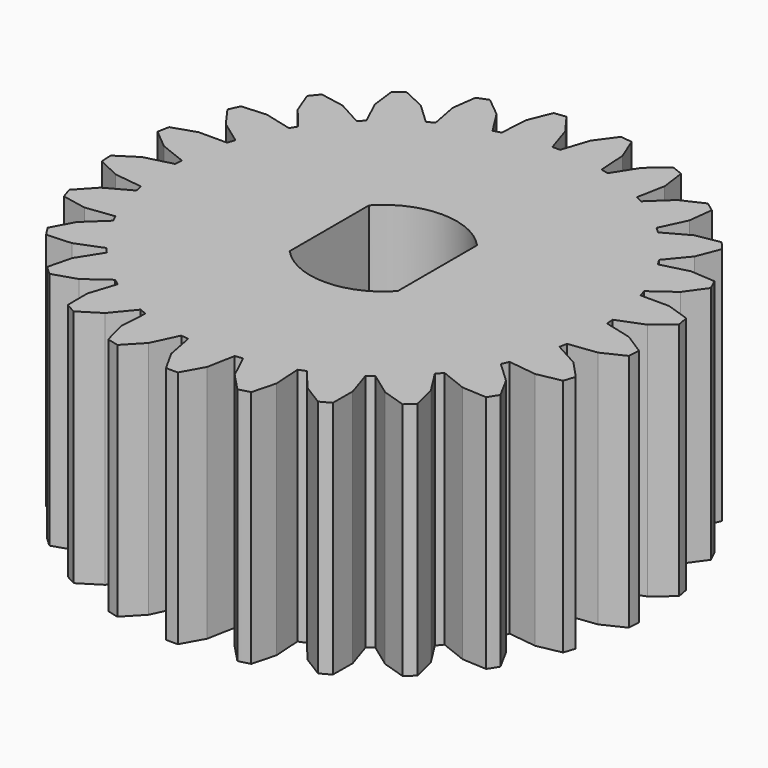
from build123d import *

# Parameters (mm, degrees)
F0_R     = 6.85
F1_DEPTH = 6.2
F3_DEPTH = 25


with BuildPart() as f1:
    # F0 (on Top) → F1 (new body)
    with BuildSketch(Plane.XY):
        Circle(F0_R)
        with BuildLine():
            ThreePointArc((1.4, -1.2845232579), (0, -1.9), (-1.4, -1.2845232579))
            Line((-1.4, -1.2845232579), (-1.4, 1.2845232579))
            ThreePointArc((-1.4, 1.2845232579), (0, 1.9), (1.4, 1.2845232579))
            Line((1.4, 1.2845232579), (1.4, -1.2845232579))
        make_face(mode=Mode.SUBTRACT)
    extrude(amount=F1_DEPTH)

    # F2 (on face) → F3 (cut)
    with BuildSketch(Plane.XY.offset(6.2)):
        with BuildLine():
            Line((0.3280050893, 6.3), (0.7057770525, 6.8135437734))
            ThreePointArc((0.7057770525, 6.8135437734), (0, 6.85), (-0.7057770525, 6.8135437734))
            Line((-0.7057770525, 6.8135437734), (-0.3280050893, 6.3))
            Line((-0.3280050893, 6.3), (-0.1, 5.5982724904))
            ThreePointArc((-0.1, 5.5982724904), (0.0002198008, 5.5998651199), (0.100452053, 5.5996637666))
            Line((0.100452053, 5.5996637666), (0.3280050893, 6.3))
        make_face()
        with BuildLine():
            ThreePointArc((-1.0108556636, 6.7750033821), (-1.7035257271, 6.6347946537), (-2.3780632008, 6.423964151))
            Line((-2.3780632008, 6.423964151), (-1.8844464954, 6.0205023665))
            Line((-1.8844464954, 6.0205023665), (-1.4890920701, 5.3975234769))
            ThreePointArc((-1.4890920701, 5.3975234769), (-1.3924169295, 5.4239897219), (-1.2952835832, 5.4487214421))
            Line((-1.2952835832, 5.4487214421), (-1.2490460829, 6.1836454637))
            Line((-1.2490460829, 6.1836454637), (-1.0108556636, 6.7750033821))
        make_face()
        with BuildLine():
            ThreePointArc((-2.6639726008, 6.3107646115), (-3.3000126676, 6.0027007583), (-3.9009268922, 5.6307432353))
            Line((-3.9009268922, 5.6307432353), (-3.3224811976, 5.3627144274))
            Line((-3.3224811976, 5.3627144274), (-2.7846190089, 4.8576282126))
            ThreePointArc((-2.7846190089, 4.8576282126), (-2.6975629831, 4.9073051017), (-2.6096317882, 4.9554159103))
            Line((-2.6096317882, 4.9554159103), (-2.747615096, 5.6787497411))
            Line((-2.747615096, 5.6787497411), (-2.6639726008, 6.3107646115))
        make_face()
        with BuildLine():
            ThreePointArc((-4.149702342, 5.4499972911), (-4.6891476756, 4.9934350978), (-5.1786810004, 4.4837220137))
            Line((-5.1786810004, 4.4837220137), (-4.5517521871, 4.3679674182))
            Line((-4.5517521871, 4.3679674182), (-3.9051780943, 4.0125103027))
            ThreePointArc((-3.9051780943, 4.0125103027), (-3.8332112335, 4.0822764541), (-3.7600072304, 4.1507433722))
            Line((-3.7600072304, 4.1507433722), (-4.0735413477, 4.8170372873))
            Line((-4.0735413477, 4.8170372873), (-4.149702342, 5.4499972911))
        make_face()
        with BuildLine():
            ThreePointArc((-5.3746910235, 4.2467865972), (-5.7836462897, 3.6704135456), (-6.1310395355, 3.054972048))
            Line((-6.1310395355, 3.054972048), (-5.4950198464, 3.0987649518))
            Line((-5.4950198464, 3.0987649518), (-4.7803604777, 2.9152716134))
            ThreePointArc((-4.7803604777, 2.9152716134), (-4.7280047246, 3.0007433634), (-4.6741275899, 3.0852643626))
            Line((-4.6741275899, 3.0852643626), (-5.143512015, 3.6526526649))
            Line((-5.143512015, 3.6526526649), (-5.3746910235, 4.2467865972))
        make_face()
        with BuildLine():
            ThreePointArc((-6.2619681013, 2.7767346827), (-6.5147371366, 2.1167664115), (-6.6981623082, 1.4342669531))
            Line((-6.6981623082, 1.4342669531), (-6.0930151995, 1.6348556871))
            Line((-6.0930151995, 1.6348556871), (-5.3551752314, 1.6348556871))
            ThreePointArc((-5.3551752314, 1.6348556871), (-5.3257202904, 1.7306625312), (-5.2945553228, 1.8259268463))
            Line((-5.2945553228, 1.8259268463), (-5.8902969058, 2.2587584421))
            Line((-5.8902969058, 2.2587584421), (-6.2619681013, 2.7767346827))
        make_face()
        with BuildLine():
            ThreePointArc((-6.7557826934, 1.1322103161), (-6.8364830897, 0.4301150588), (-6.844414909, -0.2765584093))
            Line((-6.844414909, -0.2765584093), (-6.3081639991, 0.0682224269))
            Line((-6.3081639991, 0.0682224269), (-5.5935046304, 0.2517157653))
            ThreePointArc((-5.5935046304, 0.2517157653), (-5.5888012638, 0.3518378072), (-5.5823066727, 0.451859631))
            Line((-5.5823066727, 0.451859631), (-6.2669727791, 0.7229381192))
            Line((-6.2669727791, 0.7229381192), (-6.7557826934, 1.1322103161))
        make_face()
        with BuildLine():
            ThreePointArc((-6.8251066128, -0.5834549887), (-6.7286676675, -1.2835620049), (-6.560607749, -1.9700065898))
            Line((-6.560607749, -1.9700065898), (-6.1269476548, -1.5026974992))
            Line((-6.1269476548, -1.5026974992), (-5.480373562, -1.1472403837))
            ThreePointArc((-5.480373562, -1.1472403837), (-5.5007172996, -1.0490941802), (-5.5193011641, -0.9505995868))
            Line((-5.5193011641, -0.9505995868), (-6.2498717044, -0.8583070645))
            Line((-6.2498717044, -0.8583070645), (-6.8251066128, -0.5834549887))
        make_face()
        with BuildLine():
            ThreePointArc((-6.4655839828, -2.2624596708), (-6.1980653094, -2.9165881472), (-5.8645734759, -3.539672011))
            Line((-5.8645734759, -3.539672011), (-5.560752656, -2.979197415))
            Line((-5.560752656, -2.979197415), (-5.0228904672, -2.4741112002))
            ThreePointArc((-5.0228904672, -2.4741112002), (-5.0670030372, -2.3841077219), (-5.1094976647, -2.2933291365))
            Line((-5.1094976647, -2.2933291365), (-5.8400682051, -2.3856216588))
            Line((-5.8400682051, -2.3856216588), (-6.4655839828, -2.2624596708))
        make_face()
        with BuildLine():
            ThreePointArc((-5.6998049323, -3.799305691), (-5.278015713, -4.3663543298), (-4.800046483, -4.8869268218))
            Line((-4.800046483, -4.8869268218), (-4.6451551168, -4.2685034004))
            Line((-4.6451551168, -4.2685034004), (-4.2498006916, -3.6455245108))
            ThreePointArc((-4.2498006916, -3.6455245108), (-4.3149103389, -3.5693190073), (-4.3786456357, -3.4919603822))
            Line((-4.3786456357, -3.4919603822), (-5.0633117421, -3.7630388704))
            Line((-5.0633117421, -3.7630388704), (-5.6998049323, -3.799305691))
        make_face()
        with BuildLine():
            ThreePointArc((-4.5758861756, -5.0974273617), (-4.0263289782, -5.5417664115), (-3.4339149162, -5.9271180475))
            Line((-3.4339149162, -5.9271180475), (-3.437685398, -5.2896036187))
            Line((-3.437685398, -5.2896036187), (-3.2096803087, -4.5878761091))
            ThreePointArc((-3.2096803087, -4.5878761091), (-3.2916959548, -4.5302568525), (-3.3726671978, -4.4711789146))
            Line((-3.3726671978, -4.4711789146), (-3.9684087809, -4.9040105104))
            Line((-3.9684087809, -4.9040105104), (-4.5758861756, -5.0974273617))
        make_face()
        with BuildLine():
            ThreePointArc((-3.1644476615, -6.0752589243), (-2.5216531859, -6.3689689283), (-1.8520178461, -6.5948866478))
            Line((-1.8520178461, -6.5948866478), (-2.0142132627, -5.9783385879))
            Line((-2.0142132627, -5.9783385879), (-1.9678839078, -5.2419545785))
            ThreePointArc((-1.9678839078, -5.2419545785), (-2.0616522079, -5.2065419985), (-2.1547716761, -5.169456832))
            Line((-2.1547716761, -5.169456832), (-2.6241561012, -5.7368451343))
            Line((-2.6241561012, -5.7368451343), (-3.1644476615, -6.0752589243))
        make_face()
        with BuildLine():
            ThreePointArc((-1.5541752628, -6.6713596255), (-0.8585326499, -6.795985704), (-0.1537516835, -6.8482742658))
            Line((-0.1537516835, -6.8482742658), (-0.4641807003, -6.2914325567))
            Line((-0.4641807003, -6.2914325567), (-0.6024381235, -5.5666617631))
            ThreePointArc((-0.6024381235, -5.5666617631), (-0.7020672706, -5.5556809624), (-0.8014839253, -5.5429187647))
            Line((-0.8014839253, -5.5429187647), (-1.1150180426, -6.2092126798))
            Line((-1.1150180426, -6.2092126798), (-1.5541752628, -6.6713596255))
        make_face()
        with BuildLine():
            ThreePointArc((0.1537516835, -6.8482742658), (0.8585326499, -6.795985704), (1.5541752628, -6.6713596255))
            Line((1.5541752628, -6.6713596255), (1.1150180426, -6.2092126798))
            Line((1.1150180426, -6.2092126798), (0.8008610637, -5.5415951163))
            ThreePointArc((0.8008610637, -5.5415951163), (0.7016311354, -5.5557360591), (0.6021640081, -5.5680987259))
            Line((0.6021640081, -5.5680987259), (0.4641807003, -6.2914325567))
            Line((0.4641807003, -6.2914325567), (0.1537516835, -6.8482742658))
        make_face()
        with BuildLine():
            ThreePointArc((1.8520178461, -6.5948866478), (2.5216531859, -6.3689689283), (3.1644476615, -6.0752589243))
            Line((3.1644476615, -6.0752589243), (2.6241561012, -5.7368451343))
            Line((2.6241561012, -5.7368451343), (2.1538392049, -5.1683296679))
            ThreePointArc((2.1538392049, -5.1683296679), (2.0612434767, -5.2067038266), (1.9679757624, -5.2434145662))
            Line((1.9679757624, -5.2434145662), (2.0142132627, -5.9783385879))
            Line((2.0142132627, -5.9783385879), (1.8520178461, -6.5948866478))
        make_face()
        with BuildLine():
            ThreePointArc((3.4339149162, -5.9271180475), (4.0263289782, -5.5417664115), (4.5758861756, -5.0974273617))
            Line((4.5758861756, -5.0974273617), (3.9684087809, -4.9040105104))
            Line((3.9684087809, -4.9040105104), (3.3714837076, -4.4703190587))
            ThreePointArc((3.3714837076, -4.4703190587), (3.2913403097, -4.5305152438), (3.2101323618, -4.5892673853))
            Line((3.2101323618, -4.5892673853), (3.437685398, -5.2896036187))
            Line((3.437685398, -5.2896036187), (3.4339149162, -5.9271180475))
        make_face()
        with BuildLine():
            ThreePointArc((4.800046483, -4.8869268218), (5.278015713, -4.3663543298), (5.6998049323, -3.799305691))
            Line((5.6998049323, -3.799305691), (5.0633117421, -3.7630388704))
            Line((5.0633117421, -3.7630388704), (4.3772854895, -3.4914218623))
            ThreePointArc((4.3772854895, -3.4914218623), (4.3146301263, -3.5696577262), (4.2505845388, -3.6467596565))
            Line((4.2505845388, -3.6467596565), (4.6451551168, -4.2685034004))
            Line((4.6451551168, -4.2685034004), (4.800046483, -4.8869268218))
        make_face()
        with BuildLine():
            ThreePointArc((5.8645734759, -3.539672011), (6.1980653094, -2.9165881472), (6.4655839828, -2.2624596708))
            Line((6.4655839828, -2.2624596708), (5.8400682051, -2.3856216588))
            Line((5.8400682051, -2.3856216588), (5.1080463256, -2.2931457897))
            ThreePointArc((5.1080463256, -2.2931457897), (5.066815864, -2.3845054853), (5.0239568568, -2.4751126066))
            Line((5.0239568568, -2.4751126066), (5.560752656, -2.979197415))
            Line((5.560752656, -2.979197415), (5.8645734759, -3.539672011))
        make_face()
        with BuildLine():
            ThreePointArc((6.560607749, -1.9700065898), (6.7286676675, -1.2835620049), (6.8251066128, -0.5834549887))
            Line((6.8251066128, -0.5834549887), (6.2498717044, -0.8583070645))
            Line((6.2498717044, -0.8583070645), (5.5178498249, -0.9507829336))
            ThreePointArc((5.5178498249, -0.9507829336), (5.5006349265, -1.0495259952), (5.4816554886, -1.1479451288))
            Line((5.4816554886, -1.1479451288), (6.1269476548, -1.5026974992))
            Line((6.1269476548, -1.5026974992), (6.560607749, -1.9700065898))
        make_face()
        with BuildLine():
            ThreePointArc((6.844414909, -0.2765584093), (6.8364830897, 0.4301150588), (6.7557826934, 1.1322103161))
            Line((6.7557826934, 1.1322103161), (6.2669727791, 0.7229381192))
            Line((6.2669727791, 0.7229381192), (5.5809465265, 0.451321111))
            ThreePointArc((5.5809465265, 0.451321111), (5.5888288666, 0.3513990731), (5.5949215459, 0.2513519632))
            Line((5.5949215459, 0.2513519632), (6.3081639991, 0.0682224269))
            Line((6.3081639991, 0.0682224269), (6.844414909, -0.2765584093))
        make_face()
        with BuildLine():
            ThreePointArc((6.6981623082, 1.4342669531), (6.5147371366, 2.1167664115), (6.2619681013, 2.7767346827))
            Line((6.2619681013, 2.7767346827), (5.8902969058, 2.2587584421))
            Line((5.8902969058, 2.2587584421), (5.2933718326, 1.8250669903))
            ThreePointArc((5.2933718326, 1.8250669903), (5.3258561348, 1.7302444453), (5.3566381058, 1.6348556871))
            Line((5.3566381058, 1.6348556871), (6.0930151995, 1.6348556871))
            Line((6.0930151995, 1.6348556871), (6.6981623082, 1.4342669531))
        make_face()
        with BuildLine():
            ThreePointArc((6.1310395355, 3.054972048), (5.7836462897, 3.6704135456), (5.3746910235, 4.2467865972))
            Line((5.3746910235, 4.2467865972), (5.143512015, 3.6526526649))
            Line((5.143512015, 3.6526526649), (4.6731951187, 3.0841371985))
            ThreePointArc((4.6731951187, 3.0841371985), (4.7282402749, 3.0003721955), (4.7817773932, 2.9156354155))
            Line((4.7817773932, 2.9156354155), (5.4950198464, 3.0987649518))
            Line((5.4950198464, 3.0987649518), (6.1310395355, 3.054972048))
        make_face()
        with BuildLine():
            ThreePointArc((5.1786810004, 4.4837220137), (4.6891476756, 4.9934350978), (4.149702342, 5.4499972911))
            Line((4.149702342, 5.4499972911), (4.0735413477, 4.8170372873))
            Line((4.0735413477, 4.8170372873), (3.7593843688, 4.1494197239))
            ThreePointArc((3.7593843688, 4.1494197239), (3.8335316893, 4.0819755262), (3.9064600208, 4.0132150478))
            Line((3.9064600208, 4.0132150478), (4.5517521871, 4.3679674182))
            Line((4.5517521871, 4.3679674182), (5.1786810004, 4.4837220137))
        make_face()
        with BuildLine():
            ThreePointArc((3.9009268922, 5.6307432353), (3.3000126676, 6.0027007583), (2.6639726008, 6.3107646115))
            Line((2.6639726008, 6.3107646115), (2.747615096, 5.6787497411))
            Line((2.747615096, 5.6787497411), (2.6093576729, 4.9539789475))
            ThreePointArc((2.6093576729, 4.9539789475), (2.6979482089, 4.907093322), (2.7856853984, 4.8586296191))
            Line((2.7856853984, 4.8586296191), (3.3224811976, 5.3627144274))
            Line((3.3224811976, 5.3627144274), (3.9009268922, 5.6307432353))
        make_face()
        with BuildLine():
            ThreePointArc((2.3780632008, 6.423964151), (1.7035257271, 6.6347946537), (1.0108556636, 6.7750033821))
            Line((1.0108556636, 6.7750033821), (1.2490460829, 6.1836454637))
            Line((1.2490460829, 6.1836454637), (1.2953754378, 5.4472614543))
            ThreePointArc((1.2953754378, 5.4472614543), (1.3928427201, 5.4238803974), (1.4898759174, 5.3987586226))
            Line((1.4898759174, 5.3987586226), (1.8844464954, 6.0205023665))
            Line((1.8844464954, 6.0205023665), (2.3780632008, 6.423964151))
        make_face()
    extrude(amount=-F3_DEPTH, mode=Mode.SUBTRACT)


solid = f1.part
